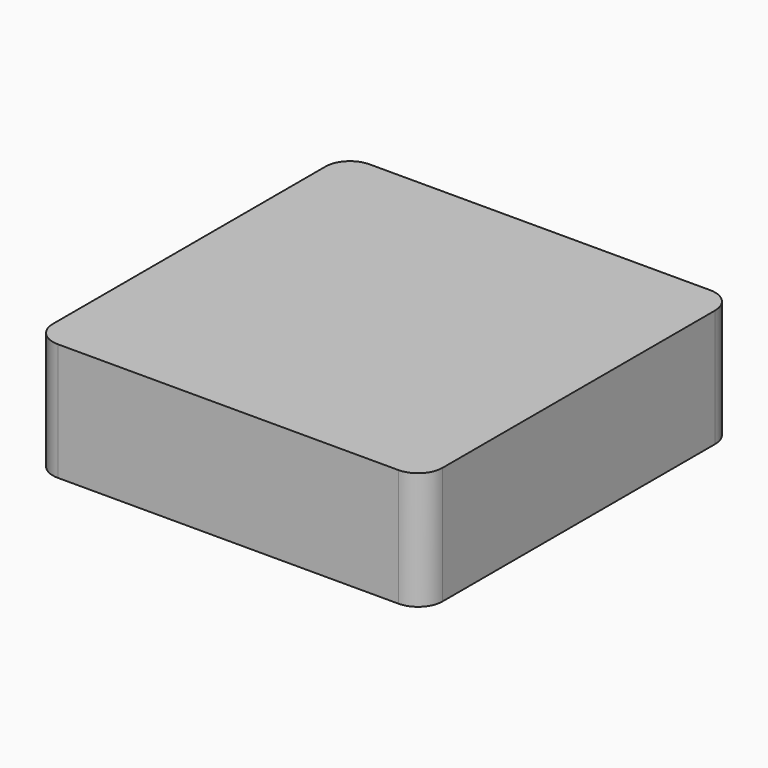
from build123d import *

# Parameters (mm, degrees)
F0_W     = 31.8
F0_H     = 31.8
F1_DEPTH = 9.6
F2_W     = 29.4
F2_H     = 29.4
F3_DEPTH = 8.4
F4_R     = 2


# Not quite as in the source:
# - a feature names something its author has since deleted; it is built from what else it names


with BuildPart() as f1:
    # F0 (on Top) → F1 (new body)
    with BuildSketch(Plane.XY):
        Rectangle(F0_W, F0_H)
    extrude(amount=F1_DEPTH)

    # F2 (on Top) → F3 (cut)
    with BuildSketch(Plane.XY):
        Rectangle(F2_W, F2_H)
    extrude(amount=F3_DEPTH, mode=Mode.SUBTRACT)

    # F4
    f4_edges = [f1.edges().sort_by_distance(p)[0] for p in [
        (-15.9, -15.9, 4.8),
        (-15.9, 15.9, 4.8),
        (15.9, 15.9, 4.8),
        (15.9, -15.9, 4.8),
    ]]
    fillet(f4_edges, radius=F4_R)


solid = f1.part
